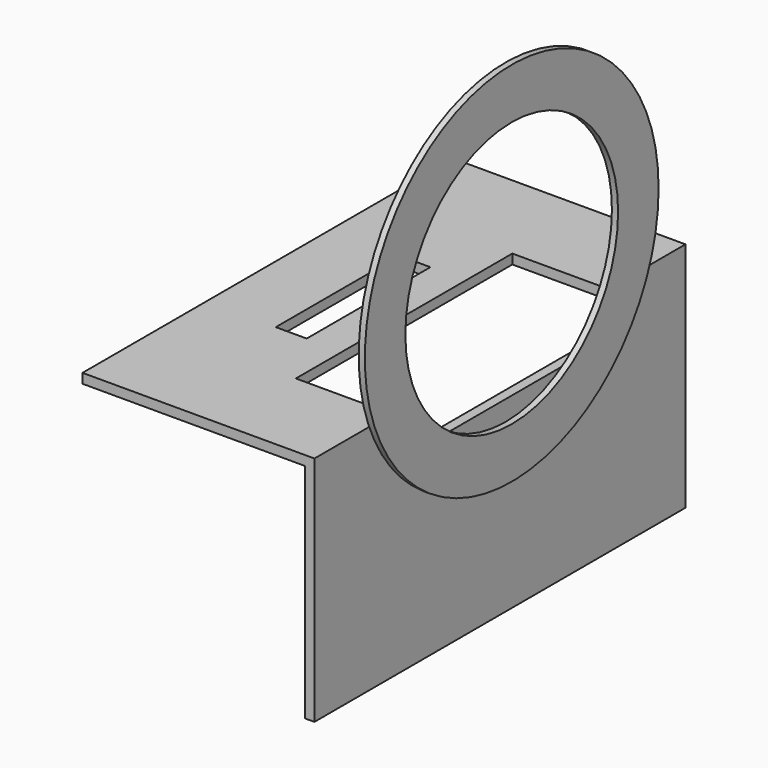
from build123d import *

# Parameters (mm, degrees)
F0_W     = 5.08
F0_H     = 25.4
F1_DEPTH = 1.5875
F3_DEPTH = 1.5875
F4_R     = 30.1625
F4_R_2   = 21.844
F5_DEPTH = 1.016


# Not quite as in the source:
# - a feature names something its author has since deleted; it is built from what else it names


with BuildPart() as f1:
    # F0 (on Top) → F1 (new body)
    with BuildSketch(Plane.XY):
        Polygon((38.1, 0), (0, 0), (0, -76.2), (38.1, -76.2), (38.1, -60.325), (22.352, -60.325), (22.352, -15.875), (38.1, -15.875), align=None)
        with Locations((13.97, -38.1)):
            Rectangle(F0_W, F0_H, mode=Mode.SUBTRACT)
    extrude(amount=F1_DEPTH)

    # F2 (on face) → F3 (join)
    with BuildSketch(Plane.YZ.offset(38.1)):
        Polygon((0, -36.5125), (0, 0), (-15.875, 0), (-15.875, -5.7785), (-60.3550081909, -5.7785), (-60.3550081909, 1.5875), (-76.2, 1.5875), (-76.2, -36.5125), align=None)
    extrude(amount=-F3_DEPTH)


with BuildPart() as f5:
    # F4 (on face) → F5 (new body)
    with BuildSketch(Plane.YZ.offset(38.1)):
        with Locations((-36.9525849819, 12.7635)):
            Circle(F4_R)
        with Locations((-36.9525849819, 12.7635)):
            Circle(F4_R_2, mode=Mode.SUBTRACT)
    extrude(amount=F5_DEPTH)


solid = Compound([f1.part, f5.part])
